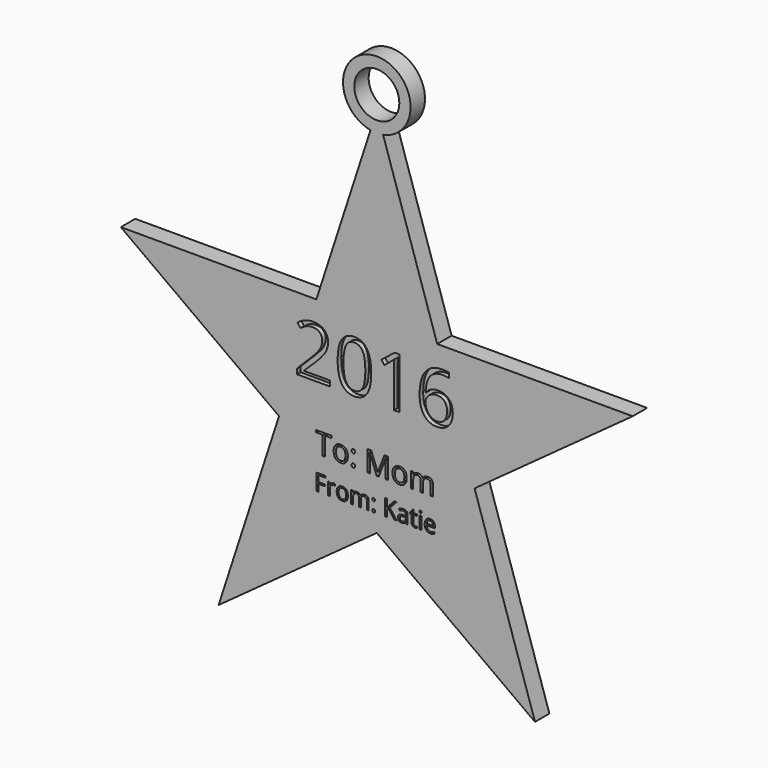
from build123d import *

# Parameters (mm, degrees)
F1_DEPTH       = 5.08
F2_TEXT_SIZE   = 6.466692624
F2_TEXT_SIZE_2 = 8.1684543855
F2_TEXT_SIZE_3 = 20.0807799249
F3_DEPTH       = 1.27
F4_R           = 9.525
F5_DEPTH       = 5.08
F6_R           = 6.35
F7_DEPTH       = 5.08


# Not quite as in the source:
# - Text() gives the source's letters only with a copy of the font that has no kerning and outlines rounded to 1/6400 em; it was checked with that copy


with BuildPart() as f1:
    # F0 (on Front) → F1 (new body)
    with BuildSketch(Plane.XZ):
        Polygon((0, 75.8720288047), (-17.0343317866, 23.4457462984), (0, 0), (17.0343317866, 23.4457462984), align=None)
        Polygon((0, 0), (-17.0343317866, 23.4457462984), (-72.1585873993, 23.4457462984), (-27.5621278063, -8.9554781944), align=None)
        Polygon((17.0343317866, 23.4457462984), (0, 0), (27.5621278063, -8.9554781944), (72.1585873993, 23.4457462984), align=None)
        Polygon((0, -28.980536208), (0, 0), (-27.5621278063, -8.9554781944), (-44.5964595929, -61.3817607007), align=None)
        Polygon((27.5621278063, -8.9554781944), (0, 0), (0, -28.980536208), (44.5964595929, -61.3817607007), align=None)
    extrude(amount=-F1_DEPTH)

    # F2 (on Front) → F3 (cut)
    with BuildSketch(Plane.XZ):
        with Locations((-17.6438564667, -24.1377800703)):
            Text('From: Katie', F2_TEXT_SIZE, font='Open Sans', text_align=(TextAlign.LEFT, TextAlign.BOTTOM))
        with Locations((-17.15375192, -14.8257426918)):
            Text('To: Mom', F2_TEXT_SIZE_2, font='Open Sans', text_align=(TextAlign.LEFT, TextAlign.BOTTOM))
        with Locations((-23.5251436243, 3.0631704722)):
            Text('2016', F2_TEXT_SIZE_3, font='Open Sans', text_align=(TextAlign.LEFT, TextAlign.BOTTOM))
    extrude(amount=-F3_DEPTH, mode=Mode.SUBTRACT)

    # F4 (on Front) → F5 (join)
    with BuildSketch(Plane.XZ):
        with Locations((0, 79.7766670585)):
            Circle(F4_R)
    extrude(amount=-F5_DEPTH)

    # F6 (on Front) → F7 (cut)
    with BuildSketch(Plane.XZ):
        with Locations((0, 79.7766670585)):
            Circle(F6_R)
    extrude(amount=-F7_DEPTH, mode=Mode.SUBTRACT)


solid = f1.part
